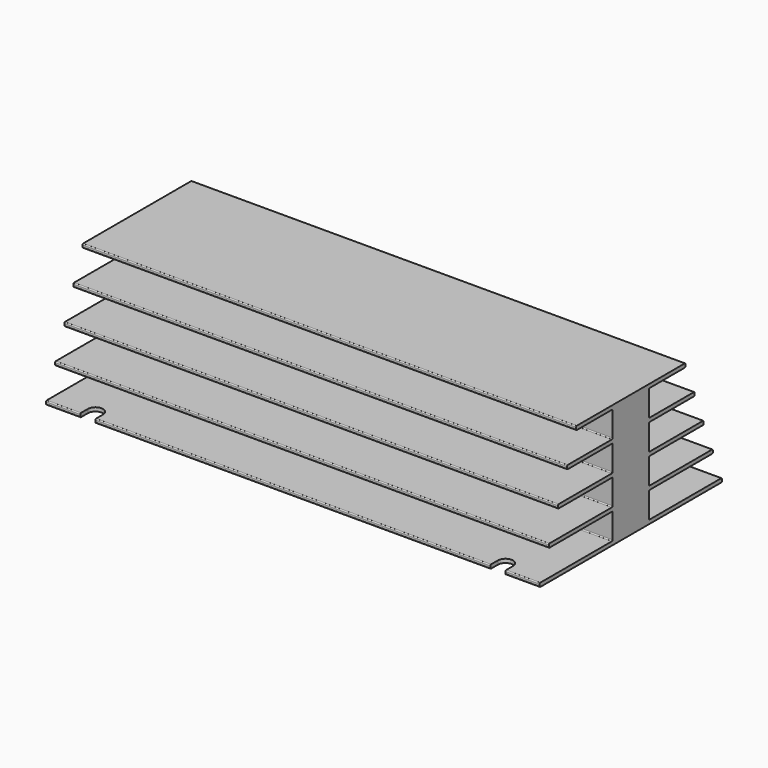
from build123d import *

# Parameters (mm, degrees)
F0_W     = 260
F0_H     = 24
F1_DEPTH = 65
F2_DEPTH = 2
F3_W     = 12
F3_H     = 2
F3_W_2   = 6
F3_W_3   = 18
F4_DEPTH = 260
F3_W_4   = 24
F3_H_2   = 13.75
F5_DEPTH = 260
F6_R     = 0.5
F7_W     = 8
F7_H     = 0.5
F7_H_2   = 4.5
F8_DEPTH = 2


# Not quite as in the source:
# - a feature names something its author has since deleted; it is built from what else it names


with BuildPart() as f1:
    # F0 (on Top) → F1 (new body)
    with BuildSketch(Plane.XY):
        with Locations((0, -24)):
            Rectangle(F0_W, F0_H)
        Rectangle(F0_W, F0_H)
        with Locations((0, 24)):
            Rectangle(F0_W, F0_H)
    extrude(amount=F1_DEPTH)

    # F0 (on Top) → F2 (join)
    with BuildSketch(Plane.XY):
        with Locations((0, -48)):
            Rectangle(F0_W, F0_H)
        with Locations((0, 48)):
            Rectangle(F0_W, F0_H)
    extrude(amount=F2_DEPTH)

    # F3 (on face) → F4 (join)
    with BuildSketch(Plane(origin=(-130, 0, 0), x_dir=(0, -1, 0), z_dir=(-1, 0, 0))):
        Polygon((36, 65), (0, 65), (0, 0), (60, 0), (60, 2), (36, 2), (12, 2), (12, 15.75), (36, 15.75), (36, 17.75), (12, 17.75), (12, 31.5), (36, 31.5), (36, 33.5), (12, 33.5), (12, 47.25), (36, 47.25), (36, 49.25), (12, 49.25), (12, 63), (36, 63), align=None)
        Polygon((0, 65), (-36, 65), (-36, 63), (-12, 63), (-12, 49.25), (-36, 49.25), (-36, 47.25), (-12, 47.25), (-12, 33.5), (-36, 33.5), (-36, 31.5), (-12, 31.5), (-12, 17.75), (-36, 17.75), (-36, 15.75), (-12, 15.75), (-12, 2), (-36, 2), (-60, 2), (-60, 0), (0, 0), align=None)
        with Locations((-42, 32.5)):
            Rectangle(F3_W, F3_H)
        with Locations((-39, 48.25)):
            Rectangle(F3_W_2, F3_H)
        with Locations((-45, 16.75)):
            Rectangle(F3_W_3, F3_H)
        with Locations((45, 16.75)):
            Rectangle(F3_W_3, F3_H)
        with Locations((42, 32.5)):
            Rectangle(F3_W, F3_H)
        with Locations((39, 48.25)):
            Rectangle(F3_W_2, F3_H)
    extrude(amount=-F4_DEPTH)

    # F3 (on face) → F5 (cut)
    with BuildSketch(Plane(origin=(-130, 0, 0), x_dir=(0, -1, 0), z_dir=(-1, 0, 0))):
        with Locations((-24, 8.875)):
            Rectangle(F3_W_4, F3_H_2)
        with Locations((-24, 56.125)):
            Rectangle(F3_W_4, F3_H_2)
        with Locations((-24, 40.375)):
            Rectangle(F3_W_4, F3_H_2)
        with Locations((-24, 24.625)):
            Rectangle(F3_W_4, F3_H_2)
        with Locations((24, 8.875)):
            Rectangle(F3_W_4, F3_H_2)
        with Locations((24, 24.625)):
            Rectangle(F3_W_4, F3_H_2)
        with Locations((24, 40.375)):
            Rectangle(F3_W_4, F3_H_2)
        with Locations((24, 56.125)):
            Rectangle(F3_W_4, F3_H_2)
    extrude(amount=-F5_DEPTH, mode=Mode.SUBTRACT)

    # F6
    f6_edges = [f1.edges().sort_by_distance(p)[0] for p in [
        (0, 36, 65),
        (0, 36, 63),
        (0, 48, 33.5),
        (0, 48, 31.5),
        (0, 54, 17.75),
        (0, 54, 15.75),
        (0, 60, 0),
        (0, 60, 2),
        (0, -60, 2),
        (0, -54, 17.75),
        (0, -48, 33.5),
        (0, -42, 49.25),
        (0, -36, 65),
        (0, -60, 0),
        (0, -54, 15.75),
        (0, -48, 31.5),
        (0, -42, 47.25),
        (0, -36, 63),
        (0, 12, 63),
        (0, 12, 49.25),
        (0, 12, 33.5),
        (0, 12, 47.25),
        (0, 12, 31.5),
        (0, 12, 15.75),
        (0, 12, 2),
        (0, -12, 63),
        (0, -12, 47.25),
        (0, -12, 31.5),
        (0, -12, 49.25),
        (0, -12, 33.5),
        (0, -12, 15.75),
        (0, -12, 17.75),
        (0, 42, 49.25),
        (0, 12, 17.75),
        (0, -12, 2),
        (0, 42, 47.25),
    ]]
    fillet(f6_edges, radius=F6_R)

    # F7 (on face) → F8 (cut)
    with BuildSketch(Plane(origin=(0, 0, 0), x_dir=(1, 0, 0), z_dir=(0, 0, -1))):
        with Locations((-108, -59.75)):
            Rectangle(F7_W, F7_H)
        with Locations((-108, -57.25)):
            Rectangle(F7_W, F7_H_2)
        with BuildLine():
            ThreePointArc((-104, -55), (-108, -51), (-112, -55))
            Line((-112, -55), (-104, -55))
        make_face()
        with Locations((-108, 59.75)):
            Rectangle(F7_W, F7_H)
        with BuildLine():
            Line((-104, 55), (-112, 55))
            ThreePointArc((-112, 55), (-108, 51), (-104, 55))
        make_face()
        with Locations((108, -59.75)):
            Rectangle(F7_W, F7_H)
        with Locations((108, -57.25)):
            Rectangle(F7_W, F7_H_2)
        with BuildLine():
            ThreePointArc((112, -55), (108, -51), (104, -55))
            Line((104, -55), (112, -55))
        make_face()
        with BuildLine():
            Line((112, 55), (104, 55))
            ThreePointArc((104, 55), (108, 51), (112, 55))
        make_face()
        with Locations((108, 59.75)):
            Rectangle(F7_W, F7_H)
        with Locations((108, 57.25)):
            Rectangle(F7_W, F7_H_2)
        with Locations((-108, 57.25)):
            Rectangle(F7_W, F7_H_2)
    extrude(amount=-F8_DEPTH, mode=Mode.SUBTRACT)


solid = f1.part
